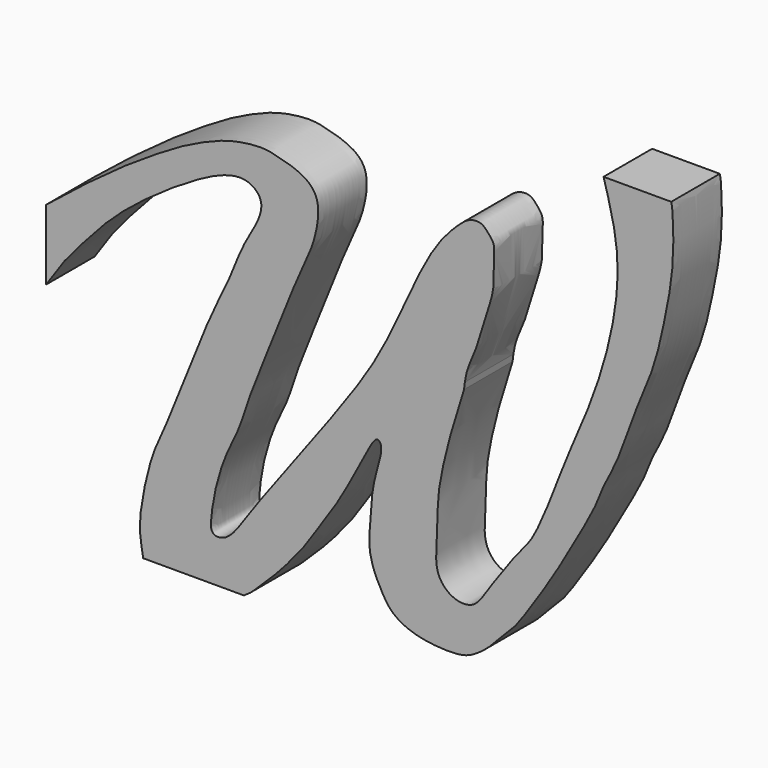
from build123d import *

# Parameters (mm, degrees)
F1_DEPTH = 25.4


with BuildPart() as f1:
    # F0 (on Front) → F1 (new body)
    with BuildSketch(Plane.XZ):
        with BuildLine():
            Line((117.0605570078, 106.2240228822), (88.7333080173, 106.2240228822))
            add(Edge.make_bspline(
                [(30.3418692201, 8.8580986485), (28.5456248688, 3.2246311971), (25.0958775577, -7.5946313262), (21.4754133945, -21.9118651221), (19.0645072916, -34.6801344898), (19.4816334182, -47.3019609408), (17.4619850954, -62.6977305166), (25.7406274861, -70.4173231157), (35.0362983923, -70.3584426579), (40.1646038888, -61.5125443559), (47.887199537, -51.1890960663), (53.6289503996, -42.6967217228), (60.2078654792, -36.8653167127), (71.6456532036, -6.4572571847), (74.0573534133, -0.2481744727), (88.4418155749, 31.2166087597), (97.3135842054, 72.7470906873), (91.2799129459, 97.322658271), (89.4260906656, 103.8024808207), (88.7333080173, 106.2240228822)],
                knots=[0, 0, 0, 0, 0.0628592493, 0.1207232891, 0.1743032514, 0.2285062179, 0.2863839478, 0.3335238533, 0.3753825281, 0.4218231019, 0.4768685014, 0.5234934226, 0.5696735125, 0.6533025189, 0.6956627685, 0.7811726076, 0.8824481009, 0.956070268, 1, 1, 1, 1], degree=3))
            add(Edge.make_bspline(
                [(30.6800070061, 11.6803441197), (30.5471132432, 10.7321565046), (30.4444912317, 9.7951275766), (30.3418692201, 8.8580986485)],
                knots=[0.9921716634, 0.9921716634, 0.9921716634, 0.9921716634, 1, 1, 1, 1], degree=3))
            add(Edge.make_bspline(
                [(-144.5774788897, 20.042611286), (-140.3361813707, 23.4753034975), (-131.3117698982, 30.7792068045), (-113.5682526455, 43.9255344567), (-101.3667302013, 51.9610158248), (-87.7205487291, 60.3646330485), (-77.805256798, 65.010535292), (-67.2288618809, 69.263818049), (-54.4464077762, 70.8434559648), (-48.3153895959, 69.5747822047), (-37.0056297212, 66.6821116529), (-28.9670429151, 59.044933082), (-32.4791153534, 41.3172664747), (-38.0855014058, 31.2196599105), (-53.3948329679, -7.8897293723), (-59.4287242613, -22.2502443249), (-63.6887306015, -36.7976268357), (-69.4257239543, -47.0181129468), (-73.7391475011, -60.5117036146), (-75.2811055028, -70.627973547), (-76.2021866945, -79.2950711355), (-68.0306569306, -79.1004454539), (-60.2502159551, -66.5346712163), (-47.5319555394, -49.753313969), (-34.8531902354, -32.4952482666), (-10.2094396384, 0.300048031), (2.3476741175, 24.6250045975), (16.0480179271, 56.6700587053), (27.6402391884, 68.5658509857), (32.3245241309, 72.430396179), (37.6566041912, 73.0517199805), (40.6480686944, 69.6326924551), (43.5122111492, 66.2091650182), (42.4020806852, 59.339544427), (43.3503106768, 49.3694465988), (38.9346042373, 38.3198006185), (36.2662357985, 26.7171546411), (31.7612771221, 17.8157176733), (30.8952906162, 13.216377477), (30.6800070061, 11.6803441197)],
                knots=[0, 0, 0, 0, 0.0306709452, 0.0652600363, 0.094061731, 0.123280002, 0.1477482557, 0.1729134495, 0.1989363533, 0.2176915695, 0.2424102006, 0.2657643004, 0.2951305199, 0.322008455, 0.3692903776, 0.3998934065, 0.4275893626, 0.4531706914, 0.48078131, 0.5052879374, 0.5245472574, 0.5413103966, 0.5691746935, 0.6031406245, 0.6380077988, 0.6847631677, 0.7249115659, 0.7683284119, 0.797842497, 0.8153853609, 0.8312553916, 0.84645477, 0.8614798665, 0.8803200008, 0.9037169066, 0.9291338239, 0.9549094134, 0.9794900107, 0.9921716634, 0.9921716634, 0.9921716634, 0.9921716634], degree=3))
            Line((-144.5774788897, 20.042611286), (-144.5774788897, -9.3671418726))
            add(Edge.make_bspline(
                [(-144.5774788897, -9.3671418726), (-141.943607797, -5.3696807148), (-136.9506047885, 2.2082663012), (-129.5613267445, 10.4855968494), (-117.6948516253, 24.07067008), (-101.3345196, 37.275043953), (-82.9905476441, 49.318741259), (-69.099869543, 56.3405034946), (-59.3460315554, 56.941566293), (-52.6892087762, 50.3435059703), (-57.2709547399, 39.703169139), (-62.4747398855, 32.0110332403), (-68.0623816194, 16.7049446235), (-72.6900325222, 8.5901078489), (-82.7941628129, -15.1448350802), (-93.0190233158, -42.5263671041), (-100.66969055, -57.2400416249), (-104.8633444074, -77.1702266269), (-105.6581149562, -87.2884741396), (-104.4852898626, -93.7856001424), (-103.909380734, -96.9759771178)],
                knots=[0, 0, 0, 0, 0.0537638318, 0.1019195566, 0.1627402543, 0.2301367836, 0.2985968706, 0.3554949699, 0.3987056898, 0.438132759, 0.4842727264, 0.5304348671, 0.5873772799, 0.6323776819, 0.7054014333, 0.7846754788, 0.8446582315, 0.9088574093, 0.9552449464, 1, 1, 1, 1], degree=3))
            Line((-103.909380734, -96.9759771178), (-61.7900043726, -96.9759771178))
            add(Edge.make_bspline(
                [(-61.7900043726, -96.9759771178), (-60.7040584224, -96.2794007928), (-58.24842892, -94.7042456259), (-53.580952397, -89.4866434426), (-48.7097393144, -85.4032850935), (-36.8262250991, -71.6982611235), (-30.9501783121, -62.1502232754), (-21.8588129031, -49.170885303), (-16.6744177891, -39.1767293272), (-10.9356641384, -28.4112777186), (-6.3257128247, -19.8719342783), (-3.6679736698, -23.3498194709), (-5.4030798636, -30.8007433424), (-8.3502467842, -40.0635677655), (-8.5160964418, -51.7825882019), (-9.86295653, -60.5615334002), (-7.9310530381, -69.3003766298), (-4.6762134316, -75.6664286316), (-0.5836627329, -83.3517040597), (8.7558072171, -88.1600999242), (19.5376575418, -89.7435953014), (28.9586623678, -89.7143328705), (34.1822722062, -87.7989379794), (40.4726276925, -83.2599999349), (45.829427762, -77.3716656502), (51.5974151047, -71.8222559753), (56.0737009488, -65.4819476003), (68.6089037128, -46.6154711249), (73.4832574008, -37.2564535259), (85.3933241871, -17.4327297431), (88.6112922033, -7.1722789059), (93.0617050174, -0.0602775728), (97.7107925265, 11.9561276699), (101.6994000836, 23.9026764666), (108.2262781474, 38.3908129201), (111.8822111978, 50.4704891516), (114.1911999859, 61.5028042999), (117.2176450611, 76.0575327354), (118.2105022734, 90.587917612), (117.7036947439, 103.3222589447), (117.2153874651, 105.52544556), (117.0605570078, 106.2240228822)],
                knots=[0, 0, 0, 0, 0.0164479877, 0.0371935305, 0.0581475246, 0.0919033128, 0.1201316363, 0.1516371479, 0.1790591714, 0.2082990266, 0.2305859946, 0.2426930754, 0.2645706844, 0.2903444894, 0.3178612388, 0.3420571144, 0.3656933015, 0.3873363886, 0.410632606, 0.4362877504, 0.4632964664, 0.4877218138, 0.5064825744, 0.5286213706, 0.5517226298, 0.5738745196, 0.5969124234, 0.6345188629, 0.6627026157, 0.7008651918, 0.7275072127, 0.7503514684, 0.7789903999, 0.8081431763, 0.8402723029, 0.8688997892, 0.8958624287, 0.9267954044, 0.9586687582, 0.9868948604, 1, 1, 1, 1], degree=3))
        make_face()
        with BuildLine():
            add(Edge.make_bspline(
                [(30.6800070061, 11.6803441197), (30.5471132432, 10.7321565046), (30.4444912317, 9.7951275766), (30.3418692201, 8.8580986485)],
                knots=[0.9921716634, 0.9921716634, 0.9921716634, 0.9921716634, 1, 1, 1, 1], degree=3))
            Line((30.3418692201, 8.8580986485), (30.6800070061, 11.6803441197))
        make_face()
    extrude(amount=F1_DEPTH)


solid = f1.part
